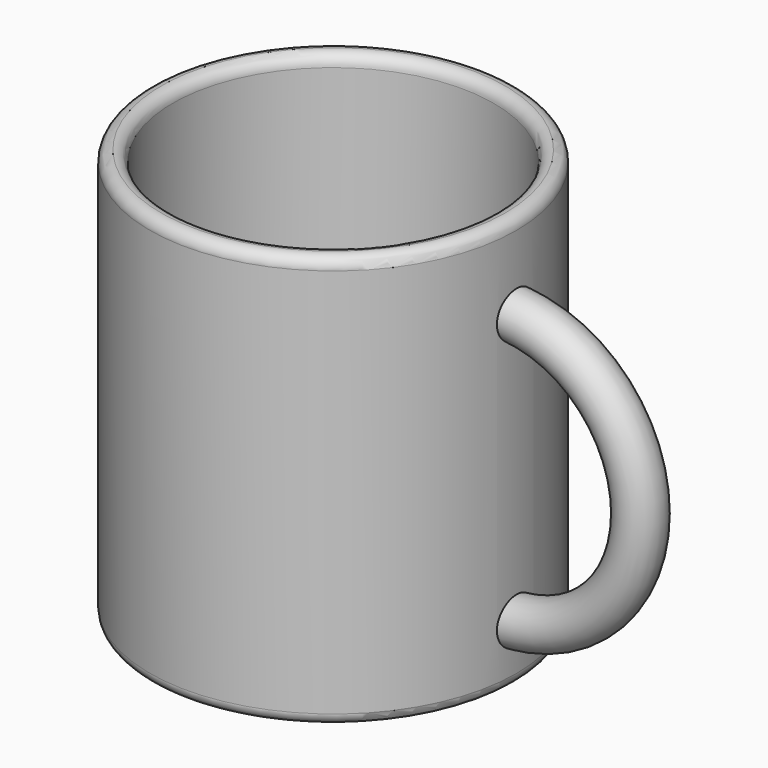
from build123d import *

# Parameters (mm, degrees)
F0_R         = 40
F1_DEPTH     = 90
F2_T         = -5
F4_R         = 5
F5_ANGLE     = 180
F6_R         = 2.49999
F7_TEXT_SIZE = 18.5813625447
F8_DEPTH     = 1.5


# Not quite as in the source:
# - a fillet or chamfer is up to 0.001 mm smaller than in the source, because OpenCascade refuses the exact size
# - Text() gives the source's letters only with a copy of the font that has no kerning and outlines rounded to 1/6400 em; it was checked with that copy


with BuildPart() as f1:
    # F0 (on Top) → F1 (new body)
    with BuildSketch(Plane.XY):
        Circle(F0_R)
    extrude(amount=F1_DEPTH)

    # F2
    f2_openings = [f1.faces().sort_by_distance(p)[0] for p in [
        (0, 0, 90),
    ]]
    offset(amount=F2_T, openings=f2_openings)

    # F4 (on offset) → F5 (revolve)
    with BuildSketch(Plane.YZ.offset(37.5)):
        with Locations((0, 71.4375004172)):
            Circle(F4_R)
    revolve(axis=Axis((37.5, 12.81696558, 41.9732145965), (0, 1, 0)), revolution_arc=F5_ANGLE)

    # F6 (radius 2.5 in the source; OpenCascade refuses exactly that, so slightly less here)
    f6_edges = [f1.edges().sort_by_distance(p)[0] for p in [
        (-40, 0, 90),
        (-35, 0, 90),
        (-40, 0, 0),
    ]]
    fillet(f6_edges, radius=F6_R)

    # F7 (on face) → F8 (cut)
    with BuildSketch(Plane(origin=(0, 0, 0), x_dir=(1, 0, 0), z_dir=(0, 0, -1))):
        with Locations((-19.307593815, -6.4362129197)):
            Text('BOY', F7_TEXT_SIZE, font='Open Sans', font_style=FontStyle.BOLDITALIC, text_align=(TextAlign.LEFT, TextAlign.BOTTOM))
    extrude(amount=-F8_DEPTH, mode=Mode.SUBTRACT)


solid = f1.part
